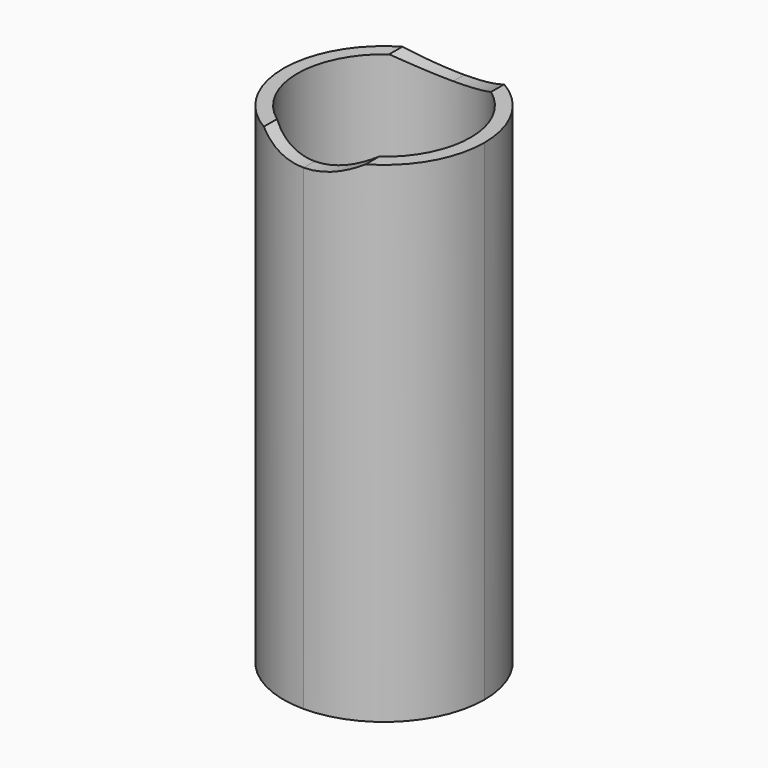
from build123d import *

# Parameters (mm, degrees)
F0_W     = 3.683
F0_H     = 3.683
F0_R     = 1.5875
F1_DEPTH = 8.98525
F3_DEPTH = 3.683
F4_R     = 1.84149


# Not quite as in the source:
# - a fillet or chamfer is up to 0.001 mm smaller than in the source, because OpenCascade refuses the exact size


with BuildPart() as f1:
    # F0 (on Top) → F1 (new body)
    with BuildSketch(Plane.XY):
        Rectangle(F0_W, F0_H)
        Circle(F0_R, mode=Mode.SUBTRACT)
    extrude(amount=F1_DEPTH)

    # F2 (on face) → F3 (cut, through all)
    with BuildSketch(Plane.XZ.offset(1.8415)):
        with BuildLine():
            Line((0, 8.98525), (-0.933255592, 8.98525))
            ThreePointArc((-0.933255592, 8.98525), (-0.4836015922, 8.7958842904), (0, 8.73125))
            Line((0, 8.73125), (0, 8.98525))
        make_face()
        with BuildLine():
            Line((0, 8.98525), (0, 8.73125))
            ThreePointArc((0, 8.73125), (0.4836015922, 8.7958842904), (0.933255592, 8.98525))
            Line((0.933255592, 8.98525), (0, 8.98525))
        make_face()
    extrude(amount=-F3_DEPTH, mode=Mode.SUBTRACT)

    # F4 (radius 1.8415 in the source; OpenCascade refuses exactly that, so slightly less here)
    f4_edges = [f1.edges().sort_by_distance(p)[0] for p in [
        (-1.8415, -1.8415, 4.492625),
        (1.8415, -1.8415, 4.492625),
        (1.8415, 1.8415, 4.492625),
        (-1.8415, 1.8415, 4.492625),
    ]]
    fillet(f4_edges, radius=F4_R)


solid = f1.part
